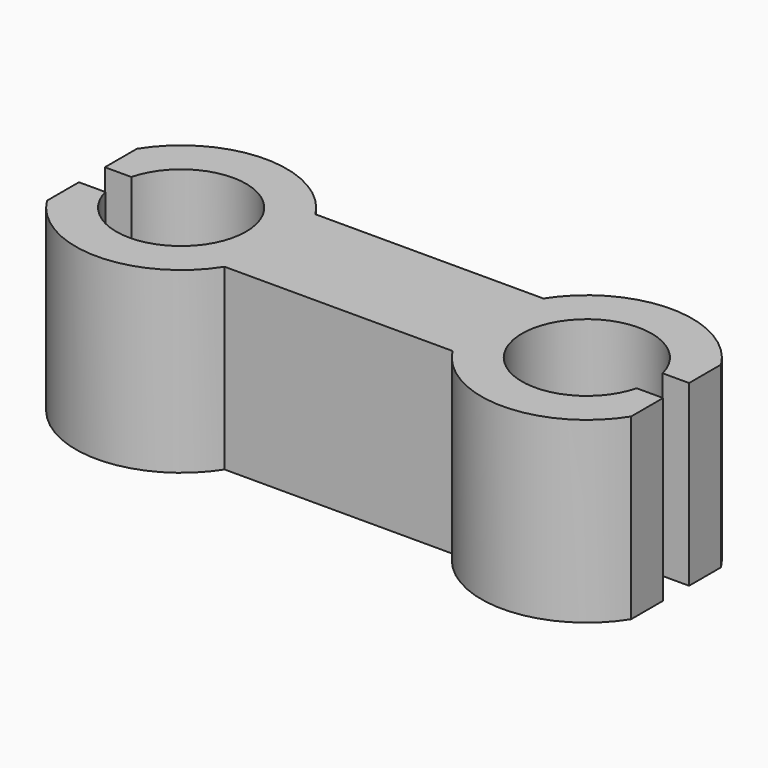
from build123d import *

# Parameters (mm, degrees)
F1_DEPTH = 11
F3_DEPTH = 11


with BuildPart() as f1:
    # F0 (on Top) → F1 (new body)
    with BuildSketch(Plane.XY):
        with BuildLine():
            Line((-12.5, 3.5), (-7.0227744249, 3.5))
            ThreePointArc((-7.0227744249, 3.5), (-19, 0), (-7.0227744249, -3.5))
            Line((-7.0227744249, -3.5), (-12.5, -3.5))
            Line((-12.5, -3.5), (-12.5, 3.5))
        make_face()
        with BuildLine():
            ThreePointArc((7.0227744249, -3.5), (6, 0), (7.0227744249, 3.5))
            Line((7.0227744249, 3.5), (-7.0227744249, 3.5))
            ThreePointArc((-7.0227744249, 3.5), (-6.2609309093, 1.8231886576), (-6, 0))
            ThreePointArc((-6, 0), (-6.2609309093, -1.8231886576), (-7.0227744249, -3.5))
            Line((-7.0227744249, -3.5), (7.0227744249, -3.5))
        make_face()
        with BuildLine():
            Line((7.0227744249, 3.5), (12.5, 3.5))
            Line((12.5, 3.5), (12.5, -3.5))
            Line((12.5, -3.5), (7.0227744249, -3.5))
            ThreePointArc((7.0227744249, -3.5), (14.3231886576, -6.2390690907), (19, 0))
            ThreePointArc((19, 0), (14.3231886576, 6.2390690907), (7.0227744249, 3.5))
        make_face()
        with BuildLine():
            ThreePointArc((-6, 0), (-6.2609309093, 1.8231886576), (-7.0227744249, 3.5))
            Line((-7.0227744249, 3.5), (-12.5, 3.5))
            Line((-12.5, 3.5), (-12.5, -3.5))
            Line((-12.5, -3.5), (-7.0227744249, -3.5))
            ThreePointArc((-7.0227744249, -3.5), (-6.2609309093, -1.8231886576), (-6, 0))
        make_face()
        with BuildLine():
            Line((12.5, -3.5), (12.5, 3.5))
            Line((12.5, 3.5), (7.0227744249, 3.5))
            ThreePointArc((7.0227744249, 3.5), (6, 0), (7.0227744249, -3.5))
            Line((7.0227744249, -3.5), (12.5, -3.5))
        make_face()
    extrude(amount=F1_DEPTH)

    # F2 (on face) → F3 (cut, through all)
    with BuildSketch(Plane.XY.offset(11)):
        with BuildLine():
            ThreePointArc((-16.3729833462, -1), (-16.5, 0), (-16.3729833462, 1))
            Line((-16.3729833462, 1), (-18, 1))
            Line((-18, 1), (-18, -1))
            Line((-18, -1), (-16.3729833462, -1))
        make_face()
        with BuildLine():
            ThreePointArc((-16.3729833462, -1), (-11.9959828301, -3.9681187851), (-8.5, 0))
            ThreePointArc((-8.5, 0), (-11.9959828301, 3.9681187851), (-16.3729833462, 1))
            Line((-16.3729833462, 1), (-16, 1))
            Line((-16, 1), (-16, -1))
            Line((-16, -1), (-16.3729833462, -1))
        make_face()
        with BuildLine():
            Line((-16, 1), (-16.3729833462, 1))
            ThreePointArc((-16.3729833462, 1), (-16.5, 0), (-16.3729833462, -1))
            Line((-16.3729833462, -1), (-16, -1))
            Line((-16, -1), (-16, 1))
        make_face()
        with BuildLine():
            ThreePointArc((16.5, 0), (16.4681187851, 0.5040171699), (16.3729833462, 1))
            Line((16.3729833462, 1), (16, 1))
            Line((16, 1), (16, -1))
            Line((16, -1), (16.3729833462, -1))
            ThreePointArc((16.3729833462, -1), (16.4681187851, -0.5040171699), (16.5, 0))
        make_face()
        with BuildLine():
            Line((18, -1), (18, 1))
            Line((18, 1), (16.3729833462, 1))
            ThreePointArc((16.3729833462, 1), (16.4681187851, 0.5040171699), (16.5, 0))
            ThreePointArc((16.5, 0), (16.4681187851, -0.5040171699), (16.3729833462, -1))
            Line((16.3729833462, -1), (18, -1))
        make_face()
        with BuildLine():
            Line((16, 1), (16.3729833462, 1))
            ThreePointArc((16.3729833462, 1), (8.5, 0), (16.3729833462, -1))
            Line((16.3729833462, -1), (16, -1))
            Line((16, -1), (16, 1))
        make_face()
        with BuildLine():
            Line((-18, -1), (-18, 1))
            Line((-18, 1), (-18.9226162893, 1))
            ThreePointArc((-18.9226162893, 1), (-19, 0), (-18.9226162893, -1))
            Line((-18.9226162893, -1), (-18, -1))
        make_face()
        with BuildLine():
            Line((18.9226162893, 1), (18, 1))
            Line((18, 1), (18, -1))
            Line((18, -1), (18.9226162893, -1))
            ThreePointArc((18.9226162893, -1), (19, 0), (18.9226162893, 1))
        make_face()
        with BuildLine():
            ThreePointArc((18.9226162893, 1), (18.5872936506, 2.2792226771), (18, 3.4641016151))
            Line((18, 3.4641016151), (18, 1))
            Line((18, 1), (18.9226162893, 1))
        make_face()
        with BuildLine():
            Line((18, -1), (18, -3.4641016151))
            ThreePointArc((18, -3.4641016151), (18.5872936506, -2.2792226771), (18.9226162893, -1))
            Line((18.9226162893, -1), (18, -1))
        make_face()
        with BuildLine():
            Line((-18.9226162893, 1), (-18, 1))
            Line((-18, 1), (-18, 3.4641016151))
            ThreePointArc((-18, 3.4641016151), (-18.5872936506, 2.2792226771), (-18.9226162893, 1))
        make_face()
        with BuildLine():
            Line((-18, -3.4641016151), (-18, -1))
            Line((-18, -1), (-18.9226162893, -1))
            ThreePointArc((-18.9226162893, -1), (-18.5872936506, -2.2792226771), (-18, -3.4641016151))
        make_face()
    extrude(amount=-F3_DEPTH, mode=Mode.SUBTRACT)


solid = f1.part
